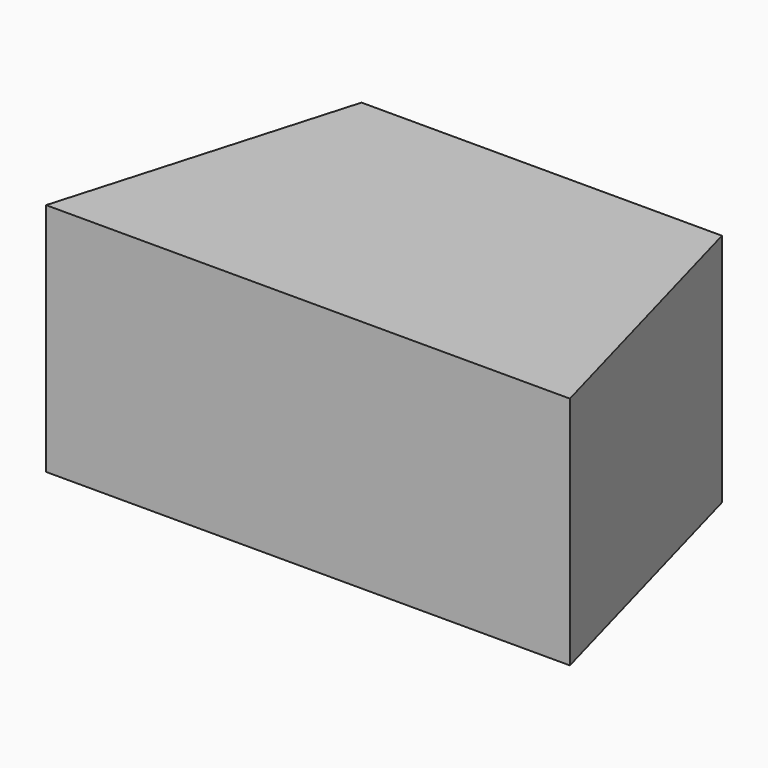
from build123d import *

# Parameters (mm, degrees)
F1_DEPTH = 30


# Not quite as in the source:
# - a feature names something its author has since deleted; it is built from what else it names


with BuildPart() as f1:
    # F0 (on Top) → F1 (new body, symmetric)
    with BuildSketch(Plane.XY):
        Polygon((46.2811469248, 34.402012825), (-45.7772985101, 34.402012825), (-67.2376081347, -39.4960939884), (66.567506886, -39.4960939884), align=None)
    extrude(amount=F1_DEPTH, both=True)


solid = f1.part
